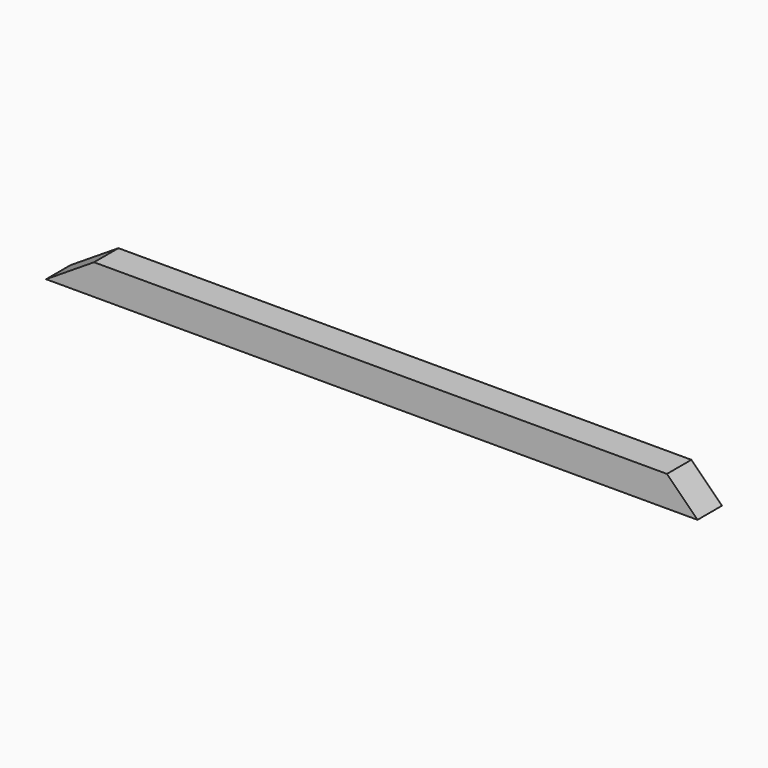
from build123d import *

# Parameters (mm, degrees)
F1_DEPTH = 19.05
F2_SIZE  = 38.09999


# Not quite as in the source:
# - a fillet or chamfer is up to 0.001 mm smaller than in the source, because OpenCascade refuses the exact size


with BuildPart() as f1:
    # F0 (on Front) → F1 (new body, symmetric)
    with BuildSketch(Plane.XZ):
        Polygon((-346.5949795118, 19.05), (-406.4, -19.05), (406.4, -19.05), (406.4, 19.05), align=None)
    extrude(amount=F1_DEPTH, both=True)

    # F2 (size 38.1 in the source; OpenCascade refuses exactly that, so slightly less here)
    f2_edges = [f1.edges().sort_by_distance(p)[0] for p in [
        (406.4, 0, 19.05),
    ]]
    chamfer(f2_edges, length=F2_SIZE)


solid = f1.part
